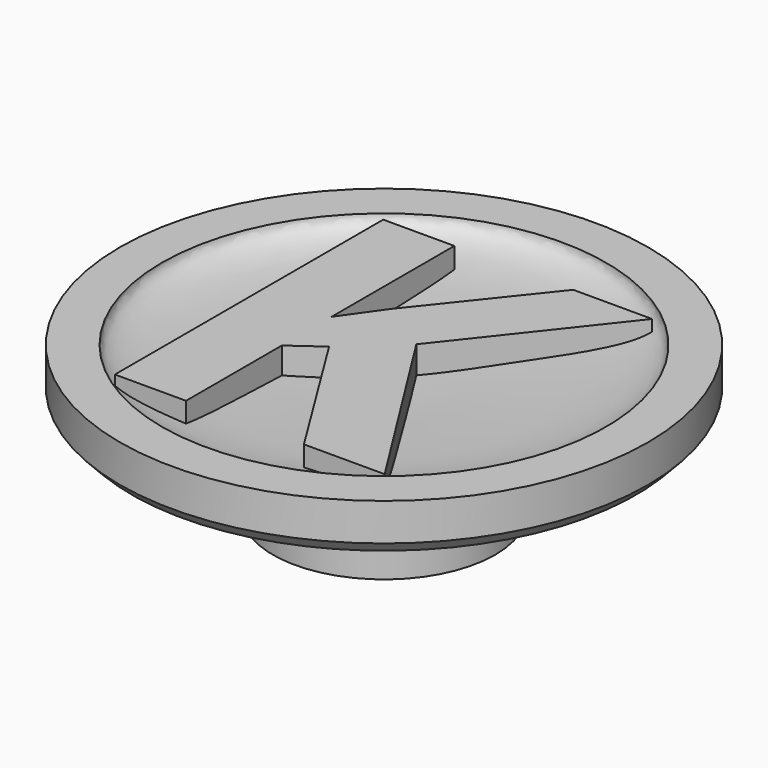
from build123d import *

# Parameters (mm, degrees)
F2_R         = 4
F3_DEPTH     = 3.55
F4_TEXT_SIZE = 16.8996212828
F5_DEPTH     = 1


# Not quite as in the source:
# - Text() gives the source's letters only with a copy of the font that has no kerning and outlines rounded to 1/6400 em; it was checked with that copy


with BuildPart() as f1:
    # F0 (on Front) → F1 (revolve)
    with BuildSketch(Plane.XZ):
        with BuildLine():
            Line((-7.9909512838, 1.8), (-9.5, 1.8))
            Line((-9.5, 1.8), (-9.5, 0.4530665231))
            Line((-9.5, 0.4530665231), (-9.0727129846, 0))
            Line((-9.0727129846, 0), (0, 0))
            Line((0, 0), (0, 0.8538585183))
            add(Edge.make_bspline(
                [(-7.9909512838, 1.8), (-7.9899121349, 1.0455427803), (-3.5041026194, 0.9095857382), (-1.4384603626, 0.7630125275), (0, 0.8538585183)],
                knots=[0.00011585, 0.00011585, 0.00011585, 0.00011585, 0.4934360698, 1, 1, 1, 1], degree=3))
        make_face()
    revolve(axis=Axis((0, 0, 1.1966938619), (0, 0, -1)))

    # F2 (on face) → F3 (join)
    with BuildSketch(Plane(origin=(0, 0, 0), x_dir=(1, 0, 0), z_dir=(0, 0, -1))):
        Circle(F2_R)
    extrude(amount=F3_DEPTH)


with BuildPart() as f5:
    # F4 (on face) → F5 (new body)
    with BuildSketch(Plane.XY.offset(1.8)):
        with Locations((-6.2902460922, -6.1354117751)):
            Text('K', F4_TEXT_SIZE, font='Open Sans', font_style=FontStyle.BOLD, text_align=(TextAlign.LEFT, TextAlign.BOTTOM))
    extrude(amount=-F5_DEPTH)


solid = Compound([f1.part, f5.part])
